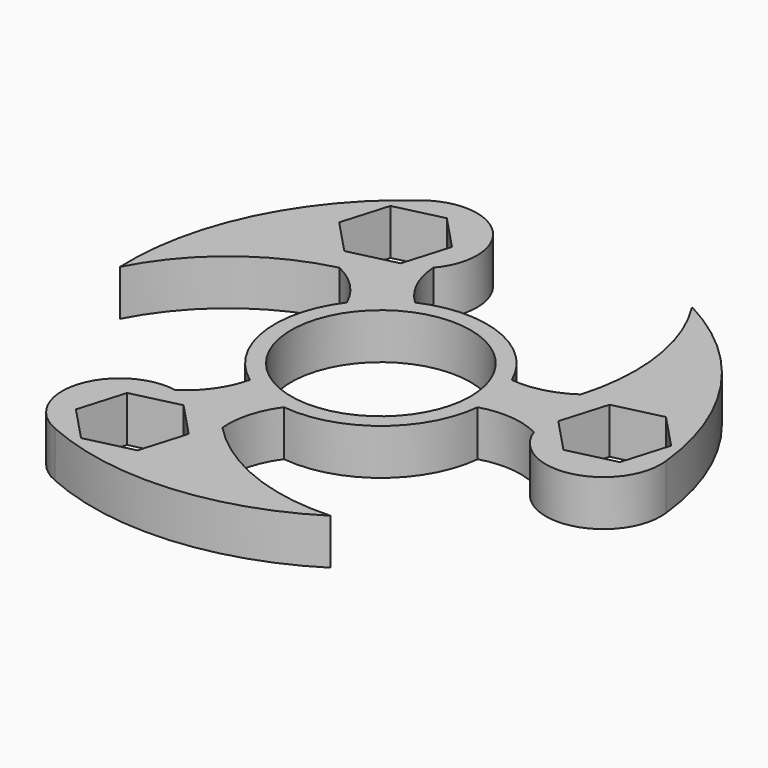
from build123d import *

# Parameters (mm, degrees)
F0_R     = 13.7215429526
F1_DEPTH = 7


# Not quite as in the source:
# - a feature names something its author has since deleted; it is built from what else it names


with BuildPart() as f1:
    # F0 (on Top) → F1 (new body)
    with BuildSketch(Plane.XY):
        with BuildLine():
            ThreePointArc((14.9110873094, 6.3741742194), (15.8866974997, 3.2532236753), (16.216368944, 0))
            ThreePointArc((16.216368944, 0), (16.1945778873, -0.8403979891), (16.1292632815, -1.6785373763))
            ThreePointArc((16.1292632815, -1.6785373763), (20.8333456957, -1.1898932874), (25.3830228197, -2.4812501212))
            ThreePointArc((25.3830228197, -2.4812501212), (35.6967714149, -8.0901996637), (42.370743035, 1.5685698162))
            ThreePointArc((42.370743035, 1.5685698162), (35.2903205619, 20.8670320083), (19.9436064757, 34.5433397021))
            ThreePointArc((19.9436064757, 34.5433397021), (24.6328655558, 21.9854776837), (23.6756761013, 8.6148816783))
            ThreePointArc((23.6756761013, 8.6148816783), (19.495827516, 6.702655598), (14.9110873094, 6.3741742194))
        make_face()
        Polygon((35.2634771892, 10.4077201887), (40.3816163825, 4.9971147515), (38.2549642206, -2.1406265287), (31.0101728654, -3.8677623716), (25.8920336721, 1.5428430657), (28.018685834, 8.6805843458), align=None, mode=Mode.SUBTRACT)
        with BuildLine():
            ThreePointArc((16.1292632815, -1.6785373763), (16.1945778873, -0.8403979891), (16.216368944, 0))
            ThreePointArc((16.216368944, 0), (15.8866974997, 3.2532236753), (14.9110873094, 6.3741742194))
            ThreePointArc((14.9110873094, 6.3741742194), (5.9163939381, 15.0985729292), (-6.6109756317, 14.8076204343))
            ThreePointArc((-6.6109756317, 14.8076204343), (-10.1175507485, 12.6730339138), (-12.9757404569, 9.7262932983))
            ThreePointArc((-12.9757404569, 9.7262932983), (-16.0339446866, -2.4255390154), (-9.5182876499, -13.129083058))
            ThreePointArc((-9.5182876499, -13.129083058), (-5.9163939381, -15.0985729292), (-1.9353468525, -16.1004675177))
            ThreePointArc((-1.9353468525, -16.1004675177), (10.1175507485, -12.6730339138), (16.1292632815, -1.6785373763))
        make_face()
        Circle(F0_R, mode=Mode.SUBTRACT)
        with BuildLine():
            ThreePointArc((-4.3771316667, -24.8111777947), (-3.9432437373, -20.2352096957), (-1.9353468525, -16.1004675177))
            ThreePointArc((-1.9353468525, -16.1004675177), (-5.9163939381, -15.0985729292), (-9.5182876499, -13.129083058))
            ThreePointArc((-9.5182876499, -13.129083058), (-11.4471506626, -17.4472599746), (-14.840337048, -20.7417175261))
            ThreePointArc((-14.840337048, -20.7417175261), (-24.8547041379, -26.8692110465), (-19.826950209, -37.4784247537))
            ThreePointArc((-19.826950209, -37.4784247537), (0.4262195398, -40.9958301185), (19.9436064757, -34.5433397021))
            ThreePointArc((19.9436064757, -34.5433397021), (6.7235494105, -32.3254261812), (-4.3771316667, -24.8111777947))
        make_face()
        Polygon((-8.6183885157, -35.742927166), (-15.8631798709, -37.4700630089), (-20.9813190642, -32.0594575716), (-18.8546669023, -24.9217162914), (-11.6098755471, -23.1945804485), (-6.4917363538, -28.6051858858), align=None, mode=Mode.SUBTRACT)
        with BuildLine():
            ThreePointArc((-12.9757404569, 9.7262932983), (-10.1175507485, 12.6730339138), (-6.6109756317, 14.8076204343))
            ThreePointArc((-6.6109756317, 14.8076204343), (-9.3861950332, 18.637153262), (-10.5426857718, 23.2229676473))
            ThreePointArc((-10.5426857718, 23.2229676473), (-10.8420672769, 34.9594107102), (-22.543792826, 35.9098549374))
            ThreePointArc((-22.543792826, 35.9098549374), (-35.7165401018, 20.1287981101), (-39.8872129515, 0))
            ThreePointArc((-39.8872129515, 0), (-31.3564149663, 10.3399484975), (-19.2985444346, 16.1962961164))
            ThreePointArc((-19.2985444346, 16.1962961164), (-15.5525837787, 13.5325540977), (-12.9757404569, 9.7262932983))
        make_face()
        Polygon((-24.5184365116, 32.4729482574), (-17.2736451565, 34.2000841003), (-12.1555059631, 28.789478663), (-14.282158125, 21.6517373829), (-21.5269494802, 19.92460154), (-26.6450886735, 25.3352069772), align=None, mode=Mode.SUBTRACT)
    extrude(amount=F1_DEPTH)


solid = f1.part
